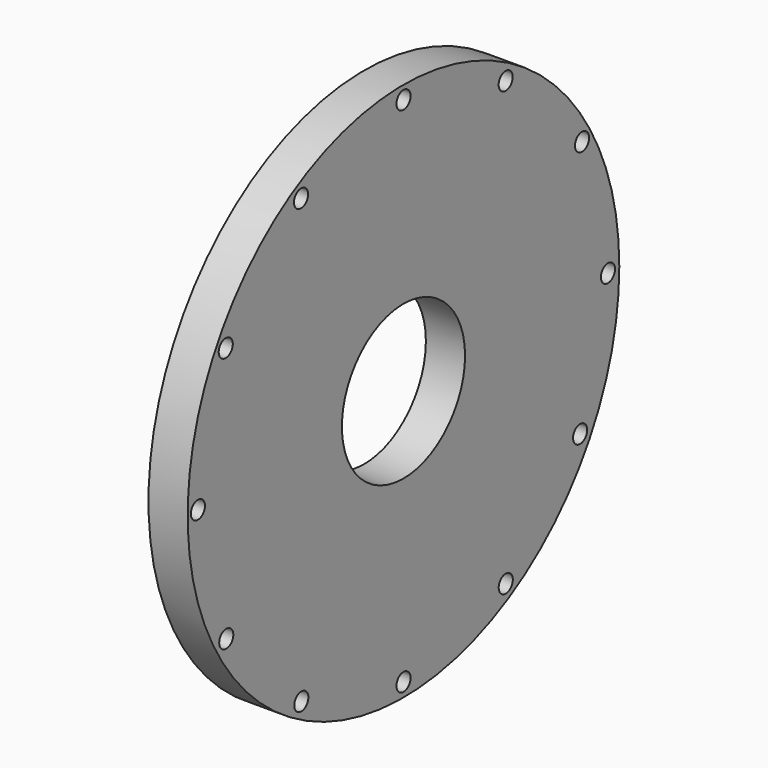
from build123d import *

# Parameters (mm, degrees)
F0_R     = 2448.457552237
F0_R_2   = 80.01
F0_R_3   = 2192.02
F0_R_4   = 698.5
F1_DEPTH = 355.6


# Not quite as in the source:
# - a feature names something its author has since deleted; it is built from what else it names


with BuildPart() as f1:
    # F0 (on Right) → F1 (new body)
    with BuildSketch(Plane.YZ):
        Circle(F0_R)
        with Locations((-1159.1256873943, -2007.6645829251)):
            Circle(F0_R_2, mode=Mode.SUBTRACT)
        with Locations((-2010.6397344548, -1160.8433919308)):
            Circle(F0_R_2, mode=Mode.SUBTRACT)
        with Locations((0, -2323.0164051056)):
            Circle(F0_R_2, mode=Mode.SUBTRACT)
        with Locations((1160.2042772772, -2009.5327554028)):
            Circle(F0_R_2, mode=Mode.SUBTRACT)
        with Locations((2003.885127001, -1156.9436174991)):
            Circle(F0_R_2, mode=Mode.SUBTRACT)
        with Locations((-2332.2319984436, 0)):
            Circle(F0_R_2, mode=Mode.SUBTRACT)
        with Locations((-2016.4296737363, 1164.1862149336)):
            Circle(F0_R_2, mode=Mode.SUBTRACT)
        with Locations((-1162.2089393996, 2013.0049320509)):
            Circle(F0_R_2, mode=Mode.SUBTRACT)
        Circle(F0_R_3, mode=Mode.SUBTRACT)
        with Locations((2319.705247879, 0)):
            Circle(F0_R_2, mode=Mode.SUBTRACT)
        with Locations((2025.6207910737, 1169.4927090025)):
            Circle(F0_R_2, mode=Mode.SUBTRACT)
        with Locations((0, 2327.2179239424)):
            Circle(F0_R_2, mode=Mode.SUBTRACT)
        with Locations((1159.3419722674, 2008.0391993142)):
            Circle(F0_R_2, mode=Mode.SUBTRACT)
        Circle(F0_R_3)
        with BuildLine():
            ThreePointArc((869.064376413, 0), (-772.1149948812, -398.8876095214), (502.8974287205, 708.7785737001))
            ThreePointArc((502.8974287205, 708.7785737001), (772.1149948812, 398.8876095214), (869.064376413, 0))
        make_face(mode=Mode.SUBTRACT)
        with BuildLine():
            ThreePointArc((869.064376413, 0), (772.1149948812, 398.8876095214), (502.8974287205, 708.7785737001))
            ThreePointArc((502.8974287205, 708.7785737001), (-772.1149948812, -398.8876095214), (869.064376413, 0))
        make_face()
        with BuildLine():
            ThreePointArc((447.4882516835, 616.764350952), (678.83357599, 346.1632217735), (762, 0))
            ThreePointArc((762, 0), (-678.83357599, -346.1632217735), (447.4882516835, 616.764350952))
        make_face(mode=Mode.SUBTRACT)
        with BuildLine():
            ThreePointArc((447.4882516835, 616.764350952), (-678.83357599, -346.1632217735), (762, 0))
            ThreePointArc((762, 0), (678.83357599, 346.1632217735), (447.4882516835, 616.764350952))
        make_face()
        Circle(F0_R_4, mode=Mode.SUBTRACT)
    extrude(amount=F1_DEPTH)


solid = f1.part
